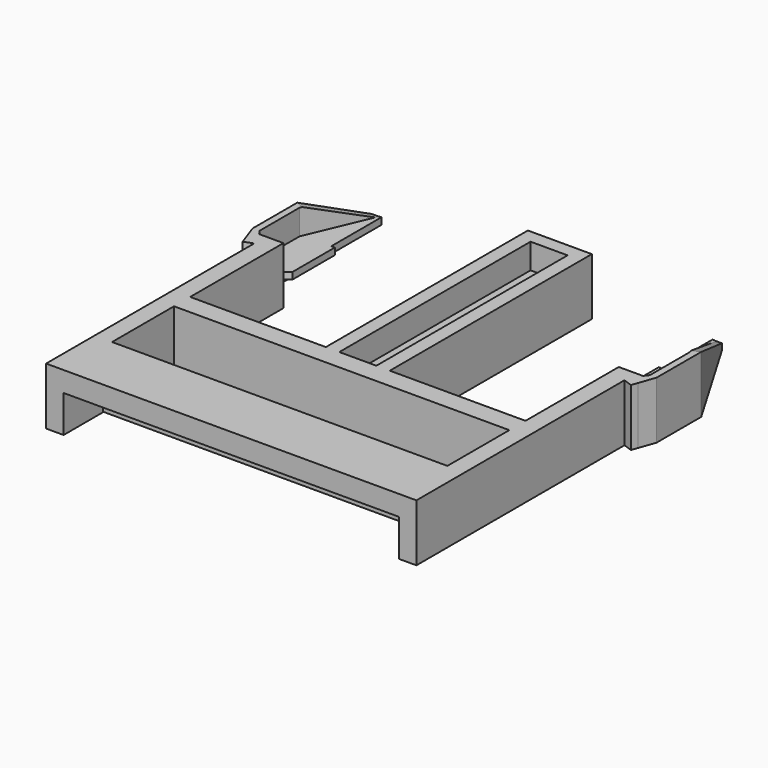
from build123d import *

# Parameters (mm, degrees)
F0_W        = 2.75
F0_H        = 35.5
F1_DEPTH    = 0.5
F2_DEPTH    = 4.25
F0_W_2      = 24.9
F0_H_2      = 3
F0_H_3      = 2.0327672064
F3_DEPTH    = 2.2
F4_T1_DEPTH = 30.8148708723
F5_W        = 9
F5_H        = 3
F6_DEPTH    = 25
F7_SIZE     = 2.99999
F8_DEPTH    = 2
F10_DEPTH   = 15
F11_DEPTH   = 25


# Not quite as in the source:
# - a fillet or chamfer that OpenCascade refuses, or shapes differently, is made with other operations: its cross-section is extruded or revolved along the edge and cut away or added
# - a fillet or chamfer is up to 0.001 mm smaller than in the source, because OpenCascade refuses the exact size


with BuildPart() as f1:
    # F0 (on Top) → F1 (new body, symmetric)
    with BuildSketch(Plane.XY):
        with Locations((1.375, 17.75)):
            Rectangle(F0_W, F0_H)
    extrude(amount=F1_DEPTH, both=True)

    # F0 (on Top) → F2 (join, symmetric)
    with BuildSketch(Plane.XY):
        Polygon((2.75, 35.5), (2.75, 0), (4.75, 0), (4.75, 37.5), (0, 37.5), (0, 35.5), align=None)
        Polygon((2.75, 0), (0, 0), (0, -3), (24.9, -3), (27.5, -3), (27.5, 0), (24.9, 0), (4.75, 0), align=None)
        Polygon((24.9, 15.6), (24.9, 0), (27.5, 0), (27.5, 15.1257448723), (27.5, 15.6), align=None)
        Polygon((27.5, -3), (24.9, -3), (24.9, -11.2172327936), (24.9, -13.25), (24.9, -16.25), (24.9, -23.5), (27.5, -23.5), align=None)
        Polygon((24.9, 17.3165686429), (24.9, 15.6), (27.5, 15.6), (29.1618686169, 15.6), (30, 17.9667025805), (30, 26.25), (25.9822437406, 35.1126976311), (24.9, 35.1126976311), (29, 25.4238011199), (29, 17.9667025805), (28.4976893067, 17.3165686429), align=None)
        Polygon((27.5, 15.6), (27.5, 15.1257448723), (28.8274421366, 14.6556516198), (29.1618686169, 15.6), align=None)
    extrude(amount=F2_DEPTH, both=True)

    # F0 (on Top) → F3 (join)
    with BuildSketch(Plane.XY):
        with Locations((12.45, -14.75)):
            Rectangle(F0_W_2, F0_H_2)
        with Locations((12.45, -12.2336163968)):
            Rectangle(F0_W_2, F0_H_3)
    extrude(amount=-F3_DEPTH)

    # F4: chamfer of 2.3 on 2 edges, made by hand

    # F4_s2 → F4_t1 (cut)
    with BuildSketch(Plane.YZ.offset(-5.9148708723)):
        Polygon((-13.95, 0), (-16.25, -2.3), (-16.25, 0), align=None)
        Polygon((-13.5172327936, 0), (-11.2172327936, -2.3), (-11.2172327936, 0), align=None)
    extrude(amount=F4_T1_DEPTH, mode=Mode.SUBTRACT)

    # F5 (on face) → F6 (join)
    with BuildSketch(Plane(origin=(24.9, 0, 0), x_dir=(0, -1, 0), z_dir=(-1, 0, 0))):
        with Locations((19, 2.75)):
            Rectangle(F5_W, F5_H)
    extrude(amount=F6_DEPTH)

    # F7 (size 3 in the source; OpenCascade refuses exactly that, so slightly less here)
    f7_edges = [f1.edges().sort_by_distance(p)[0] for p in [
        (12.4, -14.5, 1.25),
    ]]
    chamfer(f7_edges, length=F7_SIZE)

    # F8 (add): a face of the model
    f8_faces = [f1.faces().sort_by_distance(p)[0] for p in [
        (12.45, -13.7336163968, -2.2),
    ]]
    extrude(f8_faces, amount=F8_DEPTH)

    # F9 (on face) → F10 (cut)
    with BuildSketch(Plane(origin=(34.7570417343, 15.7565255862, 0), x_dir=(-0.4128877946, 0.9107818998, 0), z_dir=(0.9107818998, 0.4128877946, 0))):
        Polygon((21.2522581403, 4.25), (11.521391033, 4.25), (21.2522581403, 0.467358419), align=None)
        Polygon((21.2522581403, -0.4835649452), (11.521391033, -4.25), (21.2522581403, -4.25), align=None)
    extrude(amount=-F10_DEPTH, mode=Mode.SUBTRACT)

    # F11 (cut): faces of the model
    f11_faces = [f1.faces().sort_by_distance(p)[0] for p in [
        (25.5282194828, 34.9068733009, 2.3586792095),
        (25.5282194828, 34.9068733009, -2.3667824726),
    ]]
    extrude(f11_faces, amount=-F11_DEPTH, mode=Mode.SUBTRACT)

    # F12: F1, F1b across plane


with BuildPart() as f1b:
    # F0 (on Top) → F1, piece 2 (new body, symmetric)
    with BuildSketch(Plane.XY):
        Polygon((24.9, 35.1126976311), (24.9, 17.3165686429), (28.4976893067, 17.3165686429), (29, 17.9667025805), (29, 25.4238011199), align=None)
        Polygon((24.0585404363, 17.9667025805), (24.9, 17.3165686429), (24.9, 35.1126976311), (24.5823226869, 35.1126976311), (24.5823226869, 25.8005261421), (24.0585404363, 25.8005261421), align=None)
    extrude(amount=F1_DEPTH, both=True)


with BuildPart() as f1_1:
    add(f1.part)
    add(f1.part.mirror(Plane.YZ))
    add(f1b.part.mirror(Plane.YZ))


solid = Compound([f1b.part, f1_1.part])
